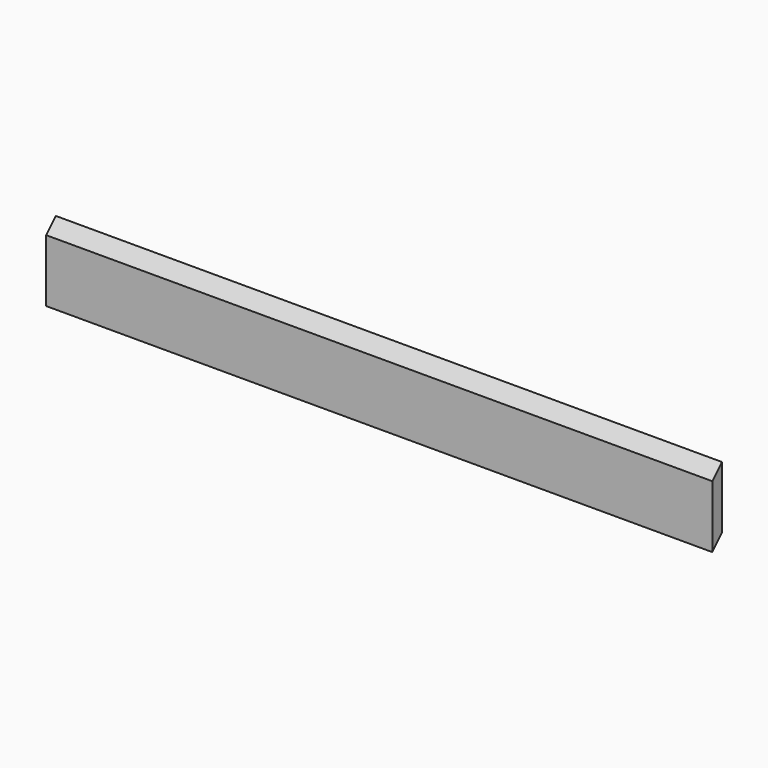
from build123d import *

# Parameters (mm, degrees)
F1_DEPTH = 527.05


# Not quite as in the source:
# - a feature of the source that left no trace in its solid (it failed there, or was rolled back) is left out


with BuildPart() as f1:
    # F0 (on Right) → F1 (new body, symmetric)
    with BuildSketch(Plane.YZ):
        Polygon((-19.05, 98.7806), (-19.05, 0), (0, 19.05), (0, 117.8306), align=None)
    extrude(amount=F1_DEPTH, both=True)


solid = f1.part
